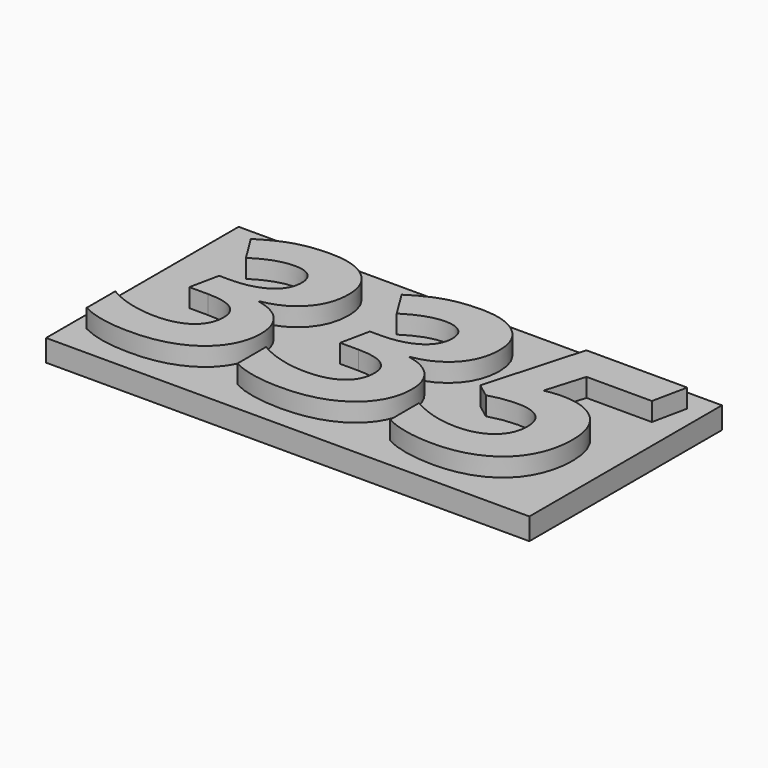
from build123d import *

# Parameters (mm, degrees)
F0_TEXT_SIZE = 127.5761932549
F1_DEPTH     = 18.796
F2_W         = 225.2210527658
F2_H         = 112.1689118445
F3_DEPTH     = 10.16


# Not quite as in the source:
# - Text() gives the source's letters only with a copy of the font that has no kerning and outlines rounded to 1/6400 em; it was checked with that copy


with BuildPart() as f1:
    # F0 (on Top) → F1 (new body)
    with BuildSketch(Plane.XY):
        with Locations((-94.1860452294, -44.3731881678)):
            Text('335', F0_TEXT_SIZE, font='Open Sans', font_style=FontStyle.BOLDITALIC, text_align=(TextAlign.LEFT, TextAlign.BOTTOM))
    extrude(amount=F1_DEPTH)


with BuildPart() as f3:
    # F2 (on Top) → F3 (new body)
    with BuildSketch(Plane.XY):
        with Locations((12.2419446707, 0.5238186568)):
            Rectangle(F2_W, F2_H)
    extrude(amount=F3_DEPTH)


solid = Compound([f1.part, f3.part])
